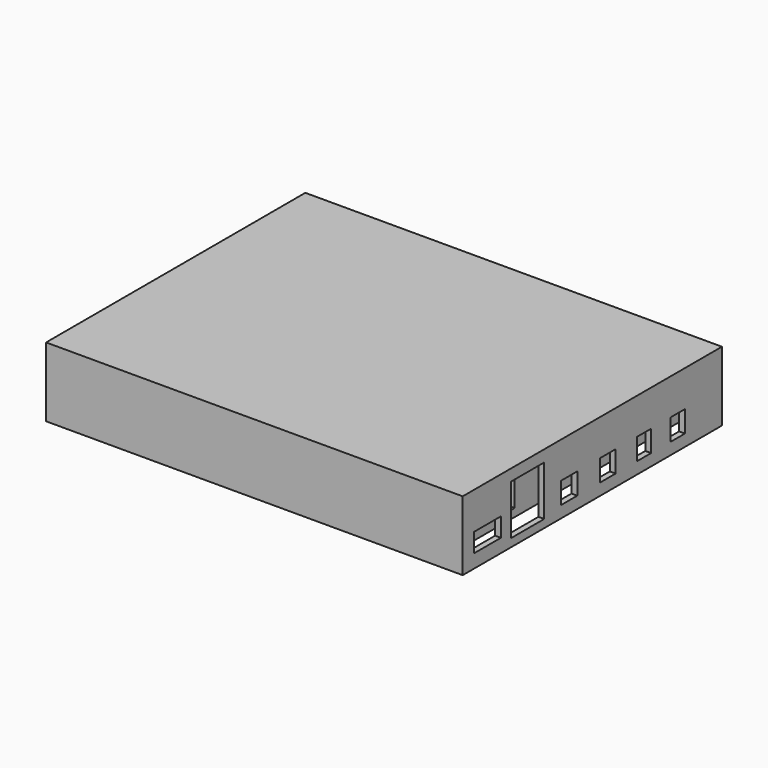
from build123d import *

# Parameters (mm, degrees)
F0_W      = 176
F0_H      = 136
F0_W_2    = 60
F0_H_2    = 60
F1_DEPTH  = 5
F2_DEPTH  = 3
F3_DEPTH  = 5
F4_DEPTH  = 3
F5_W      = 35.3965958953
F5_H      = 35.1550984732
F5_H_2    = 34.8455522954
F6_DEPTH  = 25
F7_W      = 10.2108716965
F7_H      = 14.7583791986
F7_W_2    = 5.603287369
F7_H_2    = 5.3220856935
F7_W_3    = 5.2546672523
F7_H_3    = 5.3842132911
F7_W_4    = 4.594296217
F7_H_4    = 5.3879506886
F7_W_5    = 5.3689703345
F7_H_5    = 5.0690909848
F8_DEPTH  = 5
F5_W_2    = 14.4565850496
F5_H_3    = 3.6602243781
F9_DEPTH  = 25
F5_H_4    = 3.7014111876
F5_H_5    = 5.4393112659
F10_W     = 7.6323673129
F10_H     = 15.3230233118
F10_W_2   = 7.6668392867
F11_DEPTH = 5
F12_W     = 7.3551144451
F12_H     = 17.9871618748
F12_W_2   = 7.3636993766
F13_DEPTH = 25
F14_W     = 7.5724497437
F14_H     = 17.6815595478
F14_W_2   = 7.4954973534
F14_H_2   = 17.2888860106
F15_DEPTH = 25
F16_W     = 7.9075396061
F16_H     = 17.6895577461
F17_DEPTH = 70
F18_W     = 7.6792612672
F18_H     = 9.2744342983
F18_W_2   = 8.4214285016
F18_H_2   = 9.2801470309
F18_W_3   = 7.895283401
F18_H_3   = 9.3084592372
F18_W_4   = 8.7925158441
F18_H_4   = 9.2599987984
F18_W_5   = 14.5633318461
F18_H_5   = 8.1703057513
F19_DEPTH = 5
F20_DEPTH = 25
F21_DEPTH = 25
F23_DEPTH = 2
F22_W     = 4.0043145418
F22_H     = 29.3745473027
F24_DEPTH = 4
F25_W     = 24.0477994084
F25_H     = 19.0371139906
F26_DEPTH = 10
F27_W     = 21.1675092578
F27_H     = 15.3614357114
F28_DEPTH = 25
F29_W     = 22.3702788353
F29_H     = 16.321239993
F30_DEPTH = 25


# Not quite as in the source:
# - a feature names something its author has since deleted; it is built from what else it names


with BuildPart() as f1:
    # F0 (on Top) → F1 (new body)
    with BuildSketch(Plane.XY):
        Polygon((0, 140), (0, 0), (4, 0), (4, 136), (180, 136), (180, 140), align=None)
        with Locations((92, 68)):
            Rectangle(F0_W, F0_H)
        with Locations((95.6420737505, 70)):
            Rectangle(F0_W_2, F0_H_2, mode=Mode.SUBTRACT)
        with Locations((95.6420737505, 70)):
            Rectangle(F0_W_2, F0_H_2)
        with BuildLine():
            Line((91.3972871156, 67.7366033196), (88.0402435816, 67.7366033196))
            ThreePointArc((88.0402435816, 67.7366033196), (75.9169145263, 66.5810756852), (82.7848609143, 76.6379968795))
            Line((82.7848609143, 76.6379968795), (86.1051323475, 84.5872461796))
            Line((86.1051323475, 84.5872461796), (89.6922945976, 84.5872461796))
            Line((89.6922945976, 84.5872461796), (96.8765616417, 71.4563401476))
            Line((96.8765616417, 71.4563401476), (109.4782799482, 71.4563401476))
            Line((109.4782799482, 71.4563401476), (122.3912388086, 81.5800577402))
            Line((122.3912388086, 81.5800577402), (124.4470677545, 78.9578160232))
            Line((124.4470677545, 78.9578160232), (112.5509984661, 69.6313365354))
            Line((112.5509984661, 69.6313365354), (124.4309470057, 63.2751360536))
            Line((124.4309470057, 63.2751360536), (122.3912388086, 60.2151813755))
            Line((122.3912388086, 60.2151813755), (108.6787730455, 67.7366033196))
            Line((108.6787730455, 67.7366033196), (96.5996459126, 67.7366033196))
            Line((96.5996459126, 67.7366033196), (84.0049733274, 48.6523967666))
            Line((84.0049733274, 48.6523967666), (80.3809935833, 51.0440517828))
            Line((80.3809935833, 51.0440517828), (91.3972871156, 67.7366033196))
        make_face(mode=Mode.SUBTRACT)
        with BuildLine():
            ThreePointArc((82.7848609143, 76.6379968795), (84.4233019732, 76.152156682), (85.8863730768, 75.2690073476))
            Line((85.8863730768, 75.2690073476), (87.618769124, 79.4166345349))
            Line((87.618769124, 79.4166345349), (91.5674567223, 71.4563401476))
            Line((91.5674567223, 71.4563401476), (91.3972871156, 67.7366033196))
            Line((91.3972871156, 67.7366033196), (80.3809935833, 51.0440517828))
            Line((80.3809935833, 51.0440517828), (84.0049733274, 48.6523967666))
            Line((84.0049733274, 48.6523967666), (96.5996459126, 67.7366033196))
            Line((96.5996459126, 67.7366033196), (108.6787730455, 67.7366033196))
            Line((108.6787730455, 67.7366033196), (122.3912388086, 60.2151813755))
            Line((122.3912388086, 60.2151813755), (124.4309470057, 63.2751360536))
            Line((124.4309470057, 63.2751360536), (112.5509984661, 69.6313365354))
            Line((112.5509984661, 69.6313365354), (124.4470677545, 78.9578160232))
            Line((124.4470677545, 78.9578160232), (122.3912388086, 81.5800577402))
            Line((122.3912388086, 81.5800577402), (109.4782799482, 71.4563401476))
            Line((109.4782799482, 71.4563401476), (96.8765616417, 71.4563401476))
            Line((96.8765616417, 71.4563401476), (89.6922945976, 84.5872461796))
            Line((89.6922945976, 84.5872461796), (86.1051323475, 84.5872461796))
            Line((86.1051323475, 84.5872461796), (82.7848609143, 76.6379968795))
        make_face()
        with BuildLine():
            ThreePointArc((88.0402435816, 67.7366033196), (88.3337766868, 68.8514248544), (88.432589, 70))
            ThreePointArc((88.432589, 70), (88.3925730204, 70.7325289851), (88.2730013114, 71.4563401476))
            ThreePointArc((88.2730013114, 71.4563401476), (87.4079108585, 73.5681330294), (85.8863730768, 75.2690073476))
            Line((85.8863730768, 75.2690073476), (81.7455053329, 65.3551220894))
            Line((81.7455053329, 65.3551220894), (78.6178399683, 66.6614967634))
            Line((78.6178399683, 66.6614967634), (82.7848609143, 76.6379968795))
            ThreePointArc((82.7848609143, 76.6379968795), (75.9169145263, 66.5810756852), (88.0402435816, 67.7366033196))
        make_face()
        with BuildLine():
            Line((81.7455053329, 65.3551220894), (85.8863730768, 75.2690073476))
            ThreePointArc((85.8863730768, 75.2690073476), (84.4233019732, 76.152156682), (82.7848609143, 76.6379968795))
            Line((82.7848609143, 76.6379968795), (78.6178399683, 66.6614967634))
            Line((78.6178399683, 66.6614967634), (81.7455053329, 65.3551220894))
        make_face()
        with BuildLine():
            ThreePointArc((85.8863730768, 75.2690073476), (87.4079108585, 73.5681330294), (88.2730013114, 71.4563401476))
            Line((88.2730013114, 71.4563401476), (91.5674567223, 71.4563401476))
            Line((91.5674567223, 71.4563401476), (87.618769124, 79.4166345349))
            Line((87.618769124, 79.4166345349), (85.8863730768, 75.2690073476))
        make_face()
        with BuildLine():
            ThreePointArc((88.2730013114, 71.4563401476), (88.3925730204, 70.7325289851), (88.432589, 70))
            ThreePointArc((88.432589, 70), (88.3337766868, 68.8514248544), (88.0402435816, 67.7366033196))
            Line((88.0402435816, 67.7366033196), (91.3972871156, 67.7366033196))
            Line((91.3972871156, 67.7366033196), (91.5674567223, 71.4563401476))
            Line((91.5674567223, 71.4563401476), (88.2730013114, 71.4563401476))
        make_face()
    extrude(amount=F1_DEPTH)



with BuildPart() as f2:
    # F0 (on Top) → F2 (new body)
    with BuildSketch(Plane.XY):
        with BuildLine():
            ThreePointArc((88.0402435816, 67.7366033196), (88.3337766868, 68.8514248544), (88.432589, 70))
            ThreePointArc((88.432589, 70), (88.3925730204, 70.7325289851), (88.2730013114, 71.4563401476))
            ThreePointArc((88.2730013114, 71.4563401476), (87.4079108585, 73.5681330294), (85.8863730768, 75.2690073476))
            Line((85.8863730768, 75.2690073476), (81.7455053329, 65.3551220894))
            Line((81.7455053329, 65.3551220894), (78.6178399683, 66.6614967634))
            Line((78.6178399683, 66.6614967634), (82.7848609143, 76.6379968795))
            ThreePointArc((82.7848609143, 76.6379968795), (75.9169145263, 66.5810756852), (88.0402435816, 67.7366033196))
        make_face()
    extrude(amount=-F2_DEPTH)


with BuildPart() as f3:
    # F0 (on Top) → F3 (new body)
    with BuildSketch(Plane.XY):
        with BuildLine():
            ThreePointArc((82.7848609143, 76.6379968795), (84.4233019732, 76.152156682), (85.8863730768, 75.2690073476))
            Line((85.8863730768, 75.2690073476), (87.618769124, 79.4166345349))
            Line((87.618769124, 79.4166345349), (91.5674567223, 71.4563401476))
            Line((91.5674567223, 71.4563401476), (91.3972871156, 67.7366033196))
            Line((91.3972871156, 67.7366033196), (80.3809935833, 51.0440517828))
            Line((80.3809935833, 51.0440517828), (84.0049733274, 48.6523967666))
            Line((84.0049733274, 48.6523967666), (96.5996459126, 67.7366033196))
            Line((96.5996459126, 67.7366033196), (108.6787730455, 67.7366033196))
            Line((108.6787730455, 67.7366033196), (122.3912388086, 60.2151813755))
            Line((122.3912388086, 60.2151813755), (124.4309470057, 63.2751360536))
            Line((124.4309470057, 63.2751360536), (112.5509984661, 69.6313365354))
            Line((112.5509984661, 69.6313365354), (124.4470677545, 78.9578160232))
            Line((124.4470677545, 78.9578160232), (122.3912388086, 81.5800577402))
            Line((122.3912388086, 81.5800577402), (109.4782799482, 71.4563401476))
            Line((109.4782799482, 71.4563401476), (96.8765616417, 71.4563401476))
            Line((96.8765616417, 71.4563401476), (89.6922945976, 84.5872461796))
            Line((89.6922945976, 84.5872461796), (86.1051323475, 84.5872461796))
            Line((86.1051323475, 84.5872461796), (82.7848609143, 76.6379968795))
        make_face()
        with BuildLine():
            Line((81.7455053329, 65.3551220894), (85.8863730768, 75.2690073476))
            ThreePointArc((85.8863730768, 75.2690073476), (84.4233019732, 76.152156682), (82.7848609143, 76.6379968795))
            Line((82.7848609143, 76.6379968795), (78.6178399683, 66.6614967634))
            Line((78.6178399683, 66.6614967634), (81.7455053329, 65.3551220894))
        make_face()
    extrude(amount=-F3_DEPTH)


with BuildPart() as f1_1:
    add(f1.part)

    add(f2.part)  # F4 merges F2

    add(f3.part)  # F4 merges F3
    # F0 (on Top) → F4 (join)
    with BuildSketch(Plane.XY):
        with BuildLine():
            ThreePointArc((88.2730013114, 71.4563401476), (88.3925730204, 70.7325289851), (88.432589, 70))
            ThreePointArc((88.432589, 70), (88.3337766868, 68.8514248544), (88.0402435816, 67.7366033196))
            Line((88.0402435816, 67.7366033196), (91.3972871156, 67.7366033196))
            Line((91.3972871156, 67.7366033196), (91.5674567223, 71.4563401476))
            Line((91.5674567223, 71.4563401476), (88.2730013114, 71.4563401476))
        make_face()
    extrude(amount=-F4_DEPTH)



with BuildPart() as f6:
    # F5 (on face) → F6 (new body)
    with BuildSketch(Plane(origin=(0, 0, 0), x_dir=(1, 0, 0), z_dir=(0, 0, -1))):
        Polygon((180, 0), (177.5, 0), (0, 0), (0, -140), (180, -140), align=None)
        Polygon((37.5, -137.5), (37.5, -102.5), (45, -102.5), (45, -115.5030727386), (74.5899230242, -115.5030727386), (74.5899230242, -137.5), align=None, mode=Mode.SUBTRACT)
        Polygon((45.7315295935, -102.5), (49.6945753694, -102.5), (49.6945753694, -110.0914105773), (74.5899230242, -110.0914105773), (74.5899230242, -114.6334558725), (45.7315295935, -114.6334558725), align=None, mode=Mode.SUBTRACT)
        with Locations((94.7882209718, -119.9224507634)):
            Rectangle(F5_W, F5_H, mode=Mode.SUBTRACT)
        Polygon((50, -100), (35, -100), (35, -137.5), (2.5, -137.5), (2.5, -2.5), (35.0001428115, -2.5), (35.0001428115, -40), (50, -40), align=None, mode=Mode.SUBTRACT)
        Polygon((50, -28.9151780307), (50, -37.5), (46.4391186833, -37.5), (46.4391186833, -25.8339662105), (74.5899230242, -25.8339662105), (74.5899230242, -28.9151780307), align=None, mode=Mode.SUBTRACT)
        Polygon((45, -37.5), (37.5, -37.5), (37.125878036, -2.5), (74.5899230242, -2.5), (74.5899230242, -24.3877042085), (45, -24.3877042085), align=None, mode=Mode.SUBTRACT)
        Polygon((52.5, -102.5), (52.5, -37.5), (50.6818108261, -37.5), (50.6818108261, -29.8997033387), (74.5899230242, -29.8997033387), (74.5899230242, -39.8455522954), (114.9865189195, -39.8455522954), (114.9865189195, -30.314616859), (114.9865189195, -21.8079369515), (114.9865189195, -2.5), (163.9016419649, -2.5), (167.1888530254, -2.5), (177.5, -2.5), (177.5, -137.5), (167.1888530254, -137.5), (163.9016419649, -137.5), (114.9865189195, -137.5), (114.9865189195, -118.6724507634), (114.9865189195, -110.2351546288), (114.9865189195, -99.8449015268), (74.5899230242, -99.8449015268), (74.5899230242, -109.2884466052), (50.7491268218, -109.2884466052), (50.7491268218, -102.5), align=None, mode=Mode.SUBTRACT)
        with Locations((94.7882209718, -19.9227761477)):
            Rectangle(F5_W, F5_H_2, mode=Mode.SUBTRACT)
        Polygon((167.1888530254, -2.5), (163.9016419649, -2.5), (163.9016419649, -21.8079369515), (163.9016419649, -25.4681613296), (163.9016419649, -46.3940314949), (163.9016419649, -50.0954426825), (163.9016419649, -105.1986217499), (163.9016419649, -110.6379330158), (163.9016419649, -137.5), (167.1888530254, -137.5), align=None)
    extrude(amount=F6_DEPTH)

    # F7 (on face) → F8 (cut)
    with BuildSketch(Plane.YZ.offset(52.5)):
        with Locations((70.2081844211, -7.3791895993)):
            Rectangle(F7_W, F7_H)
        with Locations((57.37423338, -11.915194802)):
            Rectangle(F7_W_2, F7_H_2)
        with Locations((47.2425129265, -11.7408647202)):
            Rectangle(F7_W_3, F7_H_3)
        with Locations((81.7268043756, -11.8016451597)):
            Rectangle(F7_W_4, F7_H_4)
        with Locations((90.9869782627, -12.1312974952)):
            Rectangle(F7_W_5, F7_H_5)
    extrude(amount=-F8_DEPTH, mode=Mode.SUBTRACT)

    # F10 (on face) → F11 (cut)
    with BuildSketch(Plane.YZ.offset(37.5)):
        with Locations((127.0232833922, -7.6615116559)):
            Rectangle(F10_W, F10_H)
        with Locations((16.000459902, -7.6615116559)):
            Rectangle(F10_W_2, F10_H)
    extrude(amount=-F11_DEPTH, mode=Mode.SUBTRACT)

    # F12 (on face) → F13 (cut)
    with BuildSketch(Plane.YZ.offset(77.0899230242)):
        with Locations((17.5473010167, -8.9935809374)):
            Rectangle(F12_W, F12_H)
        with Locations((125.3589875996, -8.9935809374)):
            Rectangle(F12_W_2, F12_H)
    extrude(amount=-F13_DEPTH, mode=Mode.SUBTRACT)

    # F14 (on face) → F15 (cut)
    with BuildSketch(Plane.YZ.offset(114.9865189195)):
        with Locations((126.9729547203, -8.8407797739)):
            Rectangle(F14_W, F14_H)
        with Locations((13.1085566245, -8.6444430053)):
            Rectangle(F14_W_2, F14_H_2)
    extrude(amount=-F15_DEPTH, mode=Mode.SUBTRACT)

    # F18 (on face) → F19 (cut)
    with BuildSketch(Plane.YZ.offset(180)):
        with Locations((97.9087017477, -15.2764413506)):
            Rectangle(F18_W, F18_H)
        with Locations((78.3716775477, -15.2735849842)):
            Rectangle(F18_W_2, F18_H_2)
        with Locations((116.0694025457, -15.2594288811)):
            Rectangle(F18_W_3, F18_H_3)
        with Locations((57.4887972325, -15.2836591005)):
            Rectangle(F18_W_4, F18_H_4)
        with Locations((13.3553545456, -15.0774200447)):
            Rectangle(F18_W_5, F18_H_5)
    extrude(amount=-F19_DEPTH, mode=Mode.SUBTRACT)


with BuildPart() as f9:
    # F5 (on face) → F9 (new body)
    with BuildSketch(Plane(origin=(0, 0, 0), x_dir=(1, 0, 0), z_dir=(0, 0, -1))):
        with Locations((156.6733494401, -23.6380491406)):
            Rectangle(F5_W_2, F5_H_3)
    extrude(amount=F9_DEPTH)


with BuildPart() as f9b:
    # F5 (on face) → F9, piece 2 (new body)
    with BuildSketch(Plane(origin=(0, 0, 0), x_dir=(1, 0, 0), z_dir=(0, 0, -1))):
        with Locations((156.6733494401, -48.2447370887)):
            Rectangle(F5_W_2, F5_H_4)
    extrude(amount=F9_DEPTH)


with BuildPart() as f9c:
    # F5 (on face) → F9, piece 3 (new body)
    with BuildSketch(Plane(origin=(0, 0, 0), x_dir=(1, 0, 0), z_dir=(0, 0, -1))):
        with Locations((156.6733494401, -107.9182773829)):
            Rectangle(F5_W_2, F5_H_5)
    extrude(amount=F9_DEPTH)


with BuildPart() as f17_tool:
    # F16 (on face) → F17 (new body)
    with BuildSketch(Plane(origin=(0, 110.6379330158, 0), x_dir=(-1, 0, 0), z_dir=(0, 1, 0))):
        with Locations((-156.5796583891, -8.844778873)):
            Rectangle(F16_W, F16_H)
    extrude(amount=-F17_DEPTH)


with BuildPart() as f9b_1:
    add(f9b.part)

    # F17: cut by f17_tool
    add(f17_tool.part, mode=Mode.SUBTRACT)


with BuildPart() as f9c_1:
    add(f9c.part)

    # F17: cut by f17_tool
    add(f17_tool.part, mode=Mode.SUBTRACT)


with BuildPart() as f1_2:
    add(f1_1.part)

    add(f6.part)  # F20 merges F6

    add(f9.part)  # F20 merges F9

    add(f9b_1.part)  # F20 merges F9b

    add(f9c_1.part)  # F20 merges F9c
    # F5 (on face) → F20 (join)
    with BuildSketch(Plane(origin=(0, 0, 0), x_dir=(1, 0, 0), z_dir=(0, 0, -1))):
        Polygon((114.9865189195, -21.8079369515), (114.9865189195, -30.314616859), (139.4990235567, -30.314616859), (139.4990235567, -110.2351546288), (114.9865189195, -110.2351546288), (114.9865189195, -118.6724507634), (149.4450569153, -118.6724507634), (149.4450569153, -110.6379330158), (149.4450569153, -105.1986217499), (149.4450569153, -50.0954426825), (149.4450569153, -46.3940314949), (149.4450569153, -25.4681613296), (149.4450569153, -21.8079369515), align=None)
    extrude(amount=F20_DEPTH)

    # F18 (on face) → F21 (cut)
    with BuildSketch(Plane.YZ.offset(180)):
        Polygon((44.034589082, 0), (41.4560027421, 0), (30.7654701173, 0), (26.2150447816, 0), (26.2150447816, -21.5090774), (44.034589082, -21.5090774), align=None)
    extrude(amount=-F21_DEPTH, mode=Mode.SUBTRACT)

    # F22 (on face) → F23 (join)
    with BuildSketch(Plane.XY):
        Polygon((156.1119556427, 97.9140773416), (149.4981348515, 97.9140773416), (149.4981348515, 92.4887284636), (153.5024493933, 92.4887284636), (153.5024493933, 63.1141811609), (149.4981348515, 63.1141811609), (149.4981348515, 58.1786595285), (156.1119556427, 58.1786595285), align=None)
    extrude(amount=-F23_DEPTH)

    # F22 (on face) → F24 (join)
    with BuildSketch(Plane.XY):
        with Locations((151.5002921224, 77.8014548123)):
            Rectangle(F22_W, F22_H)
    extrude(amount=-F24_DEPTH)

    # F25 (on face) → F26 (cut)
    with BuildSketch(Plane.YZ.offset(149.4450569153)):
        with Locations((78.0284814537, -13.5869134683)):
            Rectangle(F25_W, F25_H)
    extrude(amount=-F26_DEPTH, mode=Mode.SUBTRACT)

    # F27 (on face) → F28 (cut)
    with BuildSketch(Plane(origin=(0, 39.8455522954, 0), x_dir=(-1, 0, 0), z_dir=(0, 1, 0))):
        with Locations((-95.4313986003, -7.6807178557)):
            Rectangle(F27_W, F27_H)
    extrude(amount=-F28_DEPTH, mode=Mode.SUBTRACT)

    # F29 (on face) → F30 (cut)
    with BuildSketch(Plane.XZ.offset(-99.8449015268)):
        with Locations((94.0693542361, -8.1606199965)):
            Rectangle(F29_W, F29_H)
    extrude(amount=-F30_DEPTH, mode=Mode.SUBTRACT)


solid = f1_2.part
